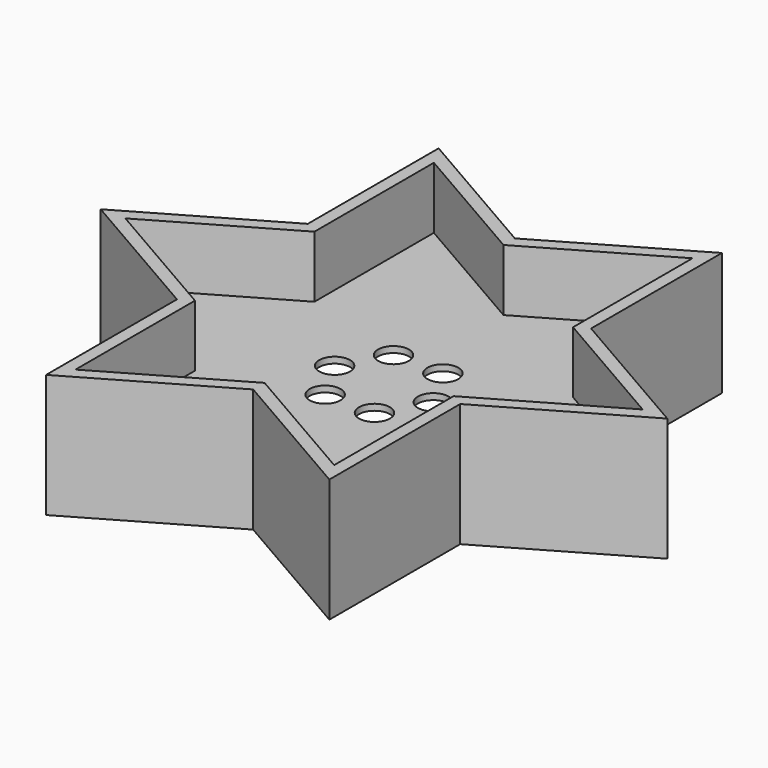
from build123d import *

# Parameters (mm, degrees)
F1_DEPTH     = 25.4
F2_T         = -2.54
F3_DEPTH     = 12.7
F4_T         = 1.27
F4_T3_DEPTH  = 27.94
F4_T5_DEPTH  = 33.2773657547
F4_T7_DEPTH  = 15.24
F4_T9_DEPTH  = 33.2773657547
F4_T11_DEPTH = 33.2773657547
F4_T13_DEPTH = 33.2773657547
F4_T15_DEPTH = 33.2773657547
F4_T17_DEPTH = 33.2773657547
F4_T19_DEPTH = 33.2773657547
F4_T21_DEPTH = 33.2773657547
F4_T23_DEPTH = 33.2773657547
F4_T25_DEPTH = 33.2773657547
F5_R         = 3.175
F6_DEPTH     = 25.4


# Not quite as in the source:
# - a shell that OpenCascade refuses in one call is made with other operations: the cavity is built on its own and cut out


with BuildPart() as f1:
    # F0 (on Top) → F1 (new body)
    with BuildSketch(Plane.XY):
        Polygon((-58.3186791779, 0), (-29.159339589, -16.8351525611), (-29.159339589, -50.5054576833), (0, -33.6703051222), (29.159339589, -50.5054576833), (29.159339589, -16.8351525611), (58.3186791779, 0), (29.159339589, 16.8351525611), (29.159339589, 50.5054576833), (0, 33.6703051222), (-29.159339589, 50.5054576833), (-29.159339589, 16.8351525611), align=None)
    extrude(amount=F1_DEPTH)

    # F2
    f2_openings = [f1.faces().sort_by_distance(p)[0] for p in [
        (0, 0, 25.4),
    ]]
    offset(amount=F2_T, openings=f2_openings, kind=Kind.INTERSECTION)

    # F0 (on Top) → F3 (join)
    with BuildSketch(Plane.XY):
        Polygon((-58.3186791779, 0), (-29.159339589, -16.8351525611), (-29.159339589, -50.5054576833), (0, -33.6703051222), (29.159339589, -50.5054576833), (29.159339589, -16.8351525611), (58.3186791779, 0), (29.159339589, 16.8351525611), (29.159339589, 50.5054576833), (0, 33.6703051222), (-29.159339589, 50.5054576833), (-29.159339589, 16.8351525611), align=None)
    extrude(amount=F3_DEPTH)

    # F4: shell of thickness 1.27, made by hand


with BuildPart() as f4_core1:
    # F4_t2: copy of F1
    add(f1.part)

    # the walls: a layer under each face that stays
    f4_faces = [f4_core1.faces().sort_by_distance(p)[0] for p in [
        (-43.7390093835, -8.4175762805, 12.7),
        (-29.159339589, -33.6703051222, 12.7),
        (-14.5796697945, -42.0878814027, 12.7),
        (14.5796697945, -42.0878814027, 12.7),
        (29.159339589, -33.6703051222, 12.7),
        (43.7390093835, -8.4175762805, 12.7),
        (43.7390093835, 8.4175762805, 12.7),
        (29.159339589, 33.6703051222, 12.7),
        (14.5796697945, 42.0878814027, 12.7),
        (-14.5796697945, 42.0878814027, 12.7),
        (-29.159339589, 33.6703051222, 12.7),
        (-54.4307672328, 0, 25.4),
        (-26.619339589, -30.7373657547, 19.05),
        (0, 0, 12.7),
        (-13.3096697945, -38.4217071934, 19.05),
        (13.3096697945, -38.4217071934, 19.05),
        (26.619339589, -30.7373657547, 19.05),
        (39.9290093835, -7.6843414387, 19.05),
        (39.9290093835, 7.6843414387, 19.05),
        (26.619339589, 30.7373657547, 19.05),
        (13.3096697945, 38.4217071934, 19.05),
        (-13.3096697945, 38.4217071934, 19.05),
        (-26.619339589, 30.7373657547, 19.05),
        (-39.9290093835, 7.6843414387, 19.05),
        (-39.9290093835, -7.6843414387, 19.05),
        (-43.7390093835, 8.4175762805, 12.7),
    ]]
    thicken(f4_faces, amount=-F4_T, mode=Mode.SUBTRACT)

    # F4_s4 → F4_t3 (cut)
    with BuildSketch(Plane.XY.offset(-1.27)):
        Polygon((-29.178389589, -16.8461510837), (-28.524339589, -15.7353002983), (-27.889339589, -16.1019177192), (-27.889339589, -16.8351525611), align=None)
        Polygon((0, -33.6923021674), (-0.635, -32.5704528594), (0, -32.2038354384), (0.635, -32.5704528594), align=None)
        Polygon((29.178389589, -16.8461510837), (27.889339589, -16.8351525611), (27.889339589, -16.1019177192), (28.524339589, -15.7353002983), align=None)
        Polygon((29.178389589, 16.8461510837), (28.524339589, 15.7353002983), (27.889339589, 16.1019177192), (27.889339589, 16.8351525611), align=None)
        Polygon((0, 33.6923021674), (0.635, 32.5704528594), (0, 32.2038354384), (-0.635, 32.5704528594), align=None)
        Polygon((-29.178389589, 16.8461510837), (-27.889339589, 16.8351525611), (-27.889339589, 16.1019177192), (-28.524339589, 15.7353002983), align=None)
    extrude(amount=F4_T3_DEPTH, mode=Mode.SUBTRACT)

    # F4_s6 → F4_t5 (cut)
    with BuildSketch(Plane.XZ.offset(14.0986828773)):
        Polygon((-26.606639589, 12.7127), (-27.889339589, 12.7), (-27.889339589, 11.43), (-26.619339589, 11.43), align=None)
        Polygon((26.606639589, 12.7127), (26.619339589, 11.43), (27.889339589, 11.43), (27.889339589, 12.7), align=None)
    extrude(amount=F4_T5_DEPTH, mode=Mode.SUBTRACT)

    # F4_s8 → F4_t7 (cut)
    with BuildSketch(Plane.XY.offset(11.43)):
        Polygon((-26.612989589, -46.0950501094), (-27.889339589, -46.106048632), (-27.889339589, -48.3057531576), (-25.984339589, -47.2059008948), align=None)
        Polygon((26.612989589, -46.0950501094), (25.984339589, -47.2059008948), (27.889339589, -48.3057531576), (27.889339589, -46.106048632), align=None)
        Polygon((53.2259791779, 0), (53.8736791779, -1.0998522628), (55.7786791779, 0), (53.8736791779, 1.0998522628), align=None)
        Polygon((26.612989589, 46.0950501094), (27.889339589, 46.106048632), (27.889339589, 48.3057531576), (25.984339589, 47.2059008948), align=None)
        Polygon((-26.612989589, 46.0950501094), (-25.984339589, 47.2059008948), (-27.889339589, 48.3057531576), (-27.889339589, 46.106048632), align=None)
        Polygon((-53.2259791779, 0), (-53.8736791779, 1.0998522628), (-55.7786791779, 0), (-53.8736791779, -1.0998522628), align=None)
    extrude(amount=F4_T7_DEPTH, mode=Mode.SUBTRACT)

    # F4_s10 → F4_t9 (cut)
    with BuildSketch(Plane(origin=(-12.2098175317, -7.0493414387, 0), x_dir=(0, 0, 1), z_dir=(-0.8660254038, -0.5, 0))):
        Polygon((12.7127, 26.606639589), (11.43, 26.619339589), (11.43, 27.889339589), (12.7, 27.889339589), align=None)
    extrude(amount=F4_T9_DEPTH, mode=Mode.SUBTRACT)

    # F4_s12 → F4_t11 (cut)
    with BuildSketch(Plane.XZ.offset(-47.376048632)):
        Polygon((-26.606639589, 12.7127), (-26.619339589, 11.43), (-27.889339589, 11.43), (-27.889339589, 12.7), align=None)
        Polygon((26.606639589, 12.7127), (26.619339589, 11.43), (27.889339589, 11.43), (27.889339589, 12.7), align=None)
    extrude(amount=F4_T11_DEPTH, mode=Mode.SUBTRACT)

    # F4_s14 → F4_t13 (cut)
    with BuildSketch(Plane(origin=(-12.2098175317, 7.0493414387, 0), x_dir=(0, 0, 1), z_dir=(-0.8660254038, 0.5, 0))):
        Polygon((12.7127, 26.606639589), (11.43, 26.619339589), (11.43, 27.889339589), (12.7, 27.889339589), align=None)
    extrude(amount=F4_T13_DEPTH, mode=Mode.SUBTRACT)

    # F4_s16 → F4_t15 (cut)
    with BuildSketch(Plane(origin=(41.0288616463, 23.688024316, 0), x_dir=(0, 0, 1), z_dir=(-0.8660254038, -0.5, 0))):
        Polygon((12.7127, 26.606639589), (11.43, 26.619339589), (11.43, 27.889339589), (12.7, 27.889339589), align=None)
    extrude(amount=F4_T15_DEPTH, mode=Mode.SUBTRACT)

    # F4_s18 → F4_t17 (cut)
    with BuildSketch(Plane(origin=(41.0288616463, -23.688024316, 0), x_dir=(0, 0, 1), z_dir=(-0.8660254038, 0.5, 0))):
        Polygon((12.7127, 26.606639589), (11.43, 26.619339589), (11.43, 27.889339589), (12.7, 27.889339589), align=None)
    extrude(amount=F4_T17_DEPTH, mode=Mode.SUBTRACT)

    # F4_s20 → F4_t19 (cut)
    with BuildSketch(Plane(origin=(12.2098175317, 7.0493414387, 0), x_dir=(0, 0, 1), z_dir=(0.8660254038, 0.5, 0))):
        Polygon((12.7127, 26.606639589), (11.43, 26.619339589), (11.43, 27.889339589), (12.7, 27.889339589), align=None)
    extrude(amount=F4_T19_DEPTH, mode=Mode.SUBTRACT)

    # F4_s22 → F4_t21 (cut)
    with BuildSketch(Plane(origin=(12.2098175317, -7.0493414387, 0), x_dir=(0, 0, 1), z_dir=(0.8660254038, -0.5, 0))):
        Polygon((12.7127, 26.606639589), (11.43, 26.619339589), (11.43, 27.889339589), (12.7, 27.889339589), align=None)
    extrude(amount=F4_T21_DEPTH, mode=Mode.SUBTRACT)

    # F4_s24 → F4_t23 (cut)
    with BuildSketch(Plane(origin=(-41.0288616463, -23.688024316, 0), x_dir=(0, 0, 1), z_dir=(0.8660254038, 0.5, 0))):
        Polygon((12.7127, 26.606639589), (11.43, 26.619339589), (11.43, 27.889339589), (12.7, 27.889339589), align=None)
    extrude(amount=F4_T23_DEPTH, mode=Mode.SUBTRACT)

    # F4_s26 → F4_t25 (cut)
    with BuildSketch(Plane(origin=(-41.0288616463, 23.688024316, 0), x_dir=(0, 0, 1), z_dir=(0.8660254038, -0.5, 0))):
        Polygon((12.7127, 26.606639589), (11.43, 26.619339589), (11.43, 27.889339589), (12.7, 27.889339589), align=None)
    extrude(amount=F4_T25_DEPTH, mode=Mode.SUBTRACT)


with BuildPart() as f1_1:
    add(f1.part)

    # what is left inside the walls is the cavity
    f4_cavity = [f4_core1.part.solids().sort_by_distance(p)[0] for p in [
        (13.94467, -8.050959, 11.4173),
    ]]
    add(f4_cavity, mode=Mode.SUBTRACT)

    # F5 (on face) → F6 (cut)
    with BuildSketch(Plane.XY.offset(12.7)):
        with Locations((5.08, 8.7988181024)):
            Circle(F5_R)
        with Locations((10.16, 0)):
            Circle(F5_R)
        with Locations((5.08, -8.7988181024)):
            Circle(F5_R)
        with Locations((-5.08, -8.7988181024)):
            Circle(F5_R)
        with Locations((-10.16, 0)):
            Circle(F5_R)
        with Locations((-5.08, 8.7988181024)):
            Circle(F5_R)
    extrude(amount=-F6_DEPTH, mode=Mode.SUBTRACT)


solid = f1_1.part
